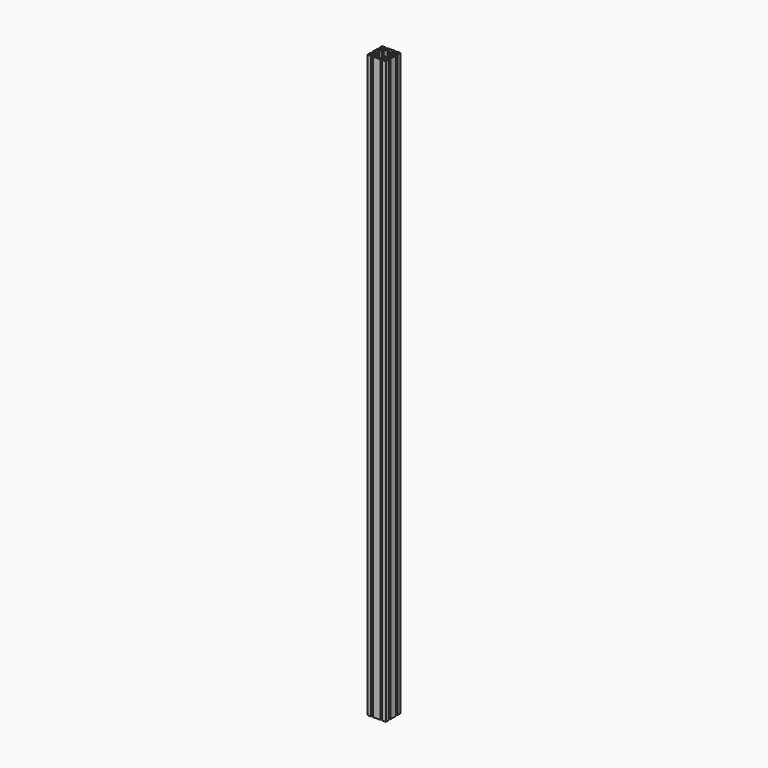
from build123d import *

# Parameters (mm, degrees)
F0_R     = 3
F0_R_2   = 2.5
F1_DEPTH = 1890
F2_R     = 2
F3_R     = 7


# Not quite as in the source:
# - a feature names something its author has since deleted; it is built from what else it names


with BuildPart() as f1:
    # F0 (on Top) → F1 (new body)
    with BuildSketch(Plane.XY):
        with BuildLine():
            Line((18.15, -30), (30, -30))
            Line((30, -30), (30, -18.15))
            Line((30, -18.15), (27.5, -18.15))
            Line((27.5, -18.15), (27.5, -20.15))
            Line((27.5, -20.15), (21.5477069044, -20.15))
            ThreePointArc((21.5477069044, -20.15), (19.5, -15), (21.5477069044, -9.85))
            Line((21.5477069044, -9.85), (27.5, -9.85))
            Line((27.5, -9.85), (27.5, -11.85))
            Line((27.5, -11.85), (30, -11.85))
            Line((30, -11.85), (30, 11.85))
            Line((30, 11.85), (27.5, 11.85))
            Line((27.5, 11.85), (27.5, 9.85))
            Line((27.5, 9.85), (21.5477069044, 9.85))
            ThreePointArc((21.5477069044, 9.85), (19.5, 15), (21.5477069044, 20.15))
            Line((21.5477069044, 20.15), (27.5, 20.15))
            Line((27.5, 20.15), (27.5, 18.15))
            Line((27.5, 18.15), (30, 18.15))
            Line((30, 18.15), (30, 30))
            Line((30, 30), (18.15, 30))
            Line((18.15, 30), (18.15, 27.5))
            Line((18.15, 27.5), (20.15, 27.5))
            Line((20.15, 27.5), (20.15, 21.5477069044))
            ThreePointArc((20.15, 21.5477069044), (15, 19.5), (9.85, 21.5477069044))
            Line((9.85, 21.5477069044), (9.85, 27.5))
            Line((9.85, 27.5), (11.85, 27.5))
            Line((11.85, 27.5), (11.85, 30))
            Line((11.85, 30), (-11.85, 30))
            Line((-11.85, 30), (-11.85, 27.5))
            Line((-11.85, 27.5), (-9.85, 27.5))
            Line((-9.85, 27.5), (-9.85, 21.5477069044))
            ThreePointArc((-9.85, 21.5477069044), (-15, 19.5), (-20.15, 21.5477069044))
            Line((-20.15, 21.5477069044), (-20.15, 27.5))
            Line((-20.15, 27.5), (-18.15, 27.5))
            Line((-18.15, 27.5), (-18.15, 30))
            Line((-18.15, 30), (-30, 30))
            Line((-30, 30), (-30, 18.15))
            Line((-30, 18.15), (-27.5, 18.15))
            Line((-27.5, 18.15), (-27.5, 20.15))
            Line((-27.5, 20.15), (-21.5477069044, 20.15))
            ThreePointArc((-21.5477069044, 20.15), (-19.5, 15), (-21.5477069044, 9.85))
            Line((-21.5477069044, 9.85), (-27.5, 9.85))
            Line((-27.5, 9.85), (-27.5, 11.85))
            Line((-27.5, 11.85), (-30, 11.85))
            Line((-30, 11.85), (-30, -11.85))
            Line((-30, -11.85), (-27.5, -11.85))
            Line((-27.5, -11.85), (-27.5, -9.85))
            Line((-27.5, -9.85), (-21.5477069044, -9.85))
            ThreePointArc((-21.5477069044, -9.85), (-19.5, -15), (-21.5477069044, -20.15))
            Line((-21.5477069044, -20.15), (-27.5, -20.15))
            Line((-27.5, -20.15), (-27.5, -18.15))
            Line((-27.5, -18.15), (-30, -18.15))
            Line((-30, -18.15), (-30, -30))
            Line((-30, -30), (-18.15, -30))
            Line((-18.15, -30), (-18.15, -27.5))
            Line((-18.15, -27.5), (-20.15, -27.5))
            Line((-20.15, -27.5), (-20.15, -21.5477069044))
            ThreePointArc((-20.15, -21.5477069044), (-15, -19.5), (-9.85, -21.5477069044))
            Line((-9.85, -21.5477069044), (-9.85, -27.5))
            Line((-9.85, -27.5), (-11.85, -27.5))
            Line((-11.85, -27.5), (-11.85, -30))
            Line((-11.85, -30), (11.85, -30))
            Line((11.85, -30), (11.85, -27.5))
            Line((11.85, -27.5), (9.85, -27.5))
            Line((9.85, -27.5), (9.85, -21.5477069044))
            ThreePointArc((9.85, -21.5477069044), (15, -19.5), (20.15, -21.5477069044))
            Line((20.15, -21.5477069044), (20.15, -27.5))
            Line((20.15, -27.5), (18.15, -27.5))
            Line((18.15, -27.5), (18.15, -30))
        make_face()
        with Locations((-25, -25)):
            Circle(F0_R, mode=Mode.SUBTRACT)
        with Locations((-15, -15)):
            Circle(F0_R_2, mode=Mode.SUBTRACT)
        with Locations((25, -25)):
            Circle(F0_R, mode=Mode.SUBTRACT)
        with Locations((15, -15)):
            Circle(F0_R_2, mode=Mode.SUBTRACT)
        with Locations((-25, 25)):
            Circle(F0_R, mode=Mode.SUBTRACT)
        with Locations((-15, 15)):
            Circle(F0_R_2, mode=Mode.SUBTRACT)
        Polygon((-7, 22), (-7, 27.5), (0, 27.5), (7, 27.5), (7, 22), (10, 16), (10, 10), (16, 10), (22, 7), (27.5, 7), (27.5, 0), (27.5, -7), (22, -7), (16, -10), (10, -10), (10, -16), (7, -22), (7, -27.5), (0, -27.5), (-7, -27.5), (-7, -22), (-10, -16), (-10, -10), (-16, -10), (-22, -7), (-27.5, -7), (-27.5, 0), (-27.5, 7), (-22, 7), (-16, 10), (-10, 10), (-10, 16), align=None, mode=Mode.SUBTRACT)
        with Locations((15, 15)):
            Circle(F0_R_2, mode=Mode.SUBTRACT)
        with Locations((25, 25)):
            Circle(F0_R, mode=Mode.SUBTRACT)
    extrude(amount=F1_DEPTH)

    # F2
    f2_edges = [f1.edges().sort_by_distance(p)[0] for p in [
        (-7, 27.5, 945),
        (7, 27.5, 945),
    ]]
    fillet(f2_edges, radius=F2_R)

    # F3
    f3_edges = [f1.edges().sort_by_distance(p)[0] for p in [
        (-10, 16, 945),
        (10, 16, 945),
    ]]
    fillet(f3_edges, radius=F3_R)


solid = f1.part
